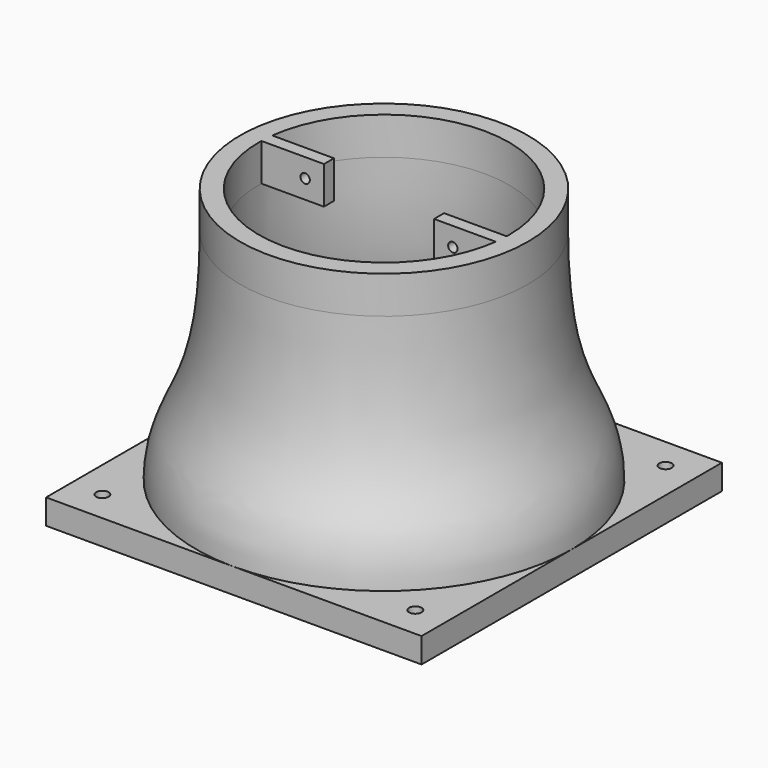
from build123d import *

# Parameters (mm, degrees)
F0_W          = 60
F0_H          = 60
F0_R          = 1
F0_R_2        = 27
F1_DEPTH      = 4
F3_R          = 23
F4_DEPTH      = 6
F5_R          = 0.75
F6_DEPTH      = 5
F6_DEPTH_BACK = 5


# Not quite as in the source:
# - the dataset's text gives a spline's control points without its knots; the knots are read off the source's solid


with BuildPart() as f1:
    # F0 (on Top) → F1 (new body)
    with BuildSketch(Plane.XY):
        Rectangle(F0_W, F0_H)
        with Locations((-25, -25)):
            Circle(F0_R, mode=Mode.SUBTRACT)
        with Locations((25, -25)):
            Circle(F0_R, mode=Mode.SUBTRACT)
        with Locations((-25, 25)):
            Circle(F0_R, mode=Mode.SUBTRACT)
        Circle(F0_R_2, mode=Mode.SUBTRACT)
        with Locations((25, 25)):
            Circle(F0_R, mode=Mode.SUBTRACT)
    extrude(amount=-F1_DEPTH)



with BuildPart() as f4:
    # F3 (on offset) → F4 (new body)
    with BuildSketch(Plane.XY.offset(35)):
        Circle(F3_R)
        with BuildLine():
            ThreePointArc((-19.843134833, 2.5), (1.2524582509, 19.9607451847), (20, 0))
            ThreePointArc((20, 0), (19.9984371947, -0.2500195366), (19.9937490231, -0.5))
            ThreePointArc((19.9937490231, -0.5), (19.9435284953, -1.5018891965), (19.843134833, -2.5))
            ThreePointArc((19.843134833, -2.5), (-1.5018891965, -19.9435284953), (-19.9937490231, 0.5))
            ThreePointArc((-19.9937490231, 0.5), (-19.9435284953, 1.5018891965), (-19.843134833, 2.5))
        make_face(mode=Mode.SUBTRACT)
        with BuildLine():
            Line((-10, 2.5), (-19.843134833, 2.5))
            ThreePointArc((-19.843134833, 2.5), (-19.9435284953, 1.5018891965), (-19.9937490231, 0.5))
            Line((-19.9937490231, 0.5), (-10, 0.5))
            Line((-10, 0.5), (-10, 2.5))
        make_face()
        with BuildLine():
            ThreePointArc((19.843134833, -2.5), (19.9435284953, -1.5018891965), (19.9937490231, -0.5))
            Line((19.9937490231, -0.5), (10, -0.5))
            Line((10, -0.5), (10, -2.5))
            Line((10, -2.5), (19.843134833, -2.5))
        make_face()
    extrude(amount=F4_DEPTH)

    # F5 (on Front) → F6 (cut, two sides)
    with BuildSketch(Plane.XZ) as f6_sk:
        with Locations((-13, 38)):
            Circle(F5_R)
        with Locations((13, 38)):
            Circle(F5_R)
    extrude(amount=-F6_DEPTH, mode=Mode.SUBTRACT)
    extrude(f6_sk.sketch, amount=F6_DEPTH_BACK, mode=Mode.SUBTRACT)


with BuildPart() as f1_1:
    add(f1.part)

    add(f4.part)  # F8 merges F4
    # F7 (on Right) → F8 (revolve)
    with BuildSketch(Plane.YZ):
        with BuildLine():
            add(Edge.make_bspline(
                [(27, 0), (27, 9.4714257866), (20, 9.4714257866), (20, 35)],
                knots=[0, 0, 0, 0, 35.6931365951, 35.6931365951, 35.6931365951, 35.6931365951], degree=3))
            Line((27, 0), (30, 0))
            add(Edge.make_bspline(
                [(30, 0), (30, 0.6843472459), (29.936581004, 1.9910917792), (29.6655509843, 3.7898301042), (29.246464382, 5.4392797223), (28.7215808007, 6.9549628049), (28.1355111863, 8.3697336208), (27.3173432912, 10.1897112488), (26.2783312641, 12.4939083516), (25.0741096829, 15.8519429796), (24.0007546171, 20.3432196278), (23.2142188638, 26.4475431113), (23, 31.8774788594), (23, 35)],
                knots=[0, 0, 0, 0, 0.0625, 0.125, 0.1875, 0.25, 0.3125, 0.375, 0.5, 0.625, 0.75, 0.875, 1, 1, 1, 1], degree=3))
            Line((23, 35), (20, 35))
        make_face()
    revolve(axis=Axis((0, 0, 13.2494084537), (0, 0, 1)))


solid = f1_1.part
